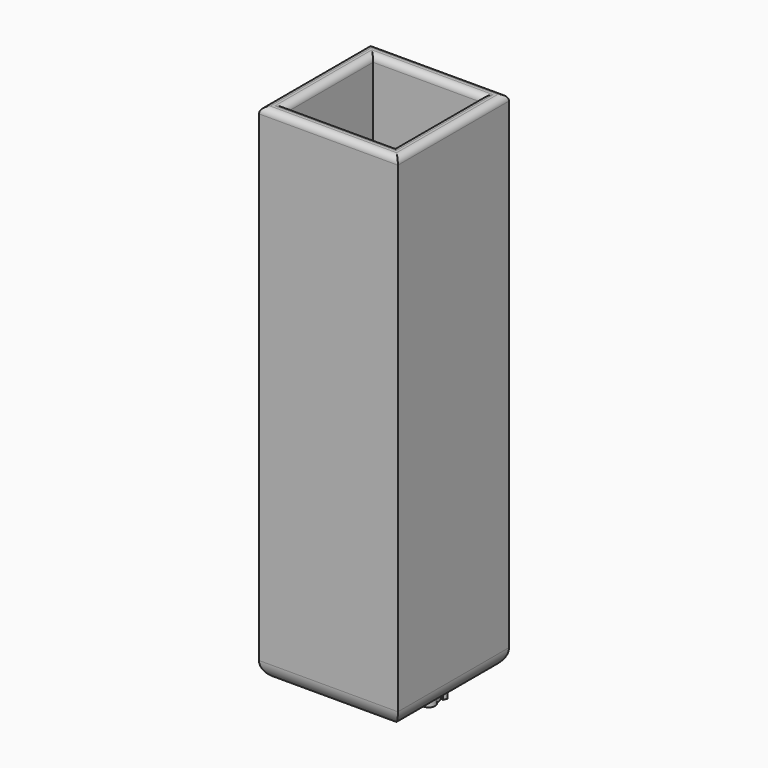
from build123d import *

# Parameters (mm, degrees)
F0_W         = 11
F0_H         = 11
F1_DEPTH     = 40
F2_W         = 8.6
F2_H         = 8.6
F3_DEPTH     = 25
F4_R         = 0.5
F5_R         = 1.4
F6_R         = 2
F7_TEXT_SIZE = 2.6055979644
F8_DEPTH     = 1


# Not quite as in the source:
# - Text() gives the source's letters only with a copy of the font that has no kerning and outlines rounded to 1/6400 em; it was checked with that copy


with BuildPart() as f1:
    # F0 (on Top) → F1 (new body)
    with BuildSketch(Plane.XY):
        Rectangle(F0_W, F0_H)
    extrude(amount=F1_DEPTH)

    # F2 (on face) → F3 (cut)
    with BuildSketch(Plane.XY.offset(40)):
        Rectangle(F2_W, F2_H)
    extrude(amount=-F3_DEPTH, mode=Mode.SUBTRACT)

    # F4
    f4_edges = [f1.edges().sort_by_distance(p)[0] for p in [
        (0, 5.5, 40),
        (5.5, 0, 40),
        (-5.5, 0, 40),
        (0, -5.5, 40),
        (0, -4.3, 40),
        (4.3, 0, 40),
        (0, 4.3, 40),
        (-4.3, 0, 40),
    ]]
    fillet(f4_edges, radius=F4_R)

    # F5
    f5_edges = [f1.edges().sort_by_distance(p)[0] for p in [
        (0, 5.5, 0),
        (-5.5, 0, 0),
        (0, -5.5, 0),
        (5.5, 0, 0),
    ]]
    fillet(f5_edges, radius=F5_R)

    # F6
    f6_edges = [f1.edges().sort_by_distance(p)[0] for p in [
        (0, -4.3, 15),
        (4.3, 0, 15),
        (0, 4.3, 15),
        (-4.3, 0, 15),
    ]]
    fillet(f6_edges, radius=F6_R)


with BuildPart() as f8:
    # F7 (on Top) → F8 (new body)
    with BuildSketch(Plane.XY):
        with Locations((-3.9, -0.3760305344)):
            Text('CiQUS', F7_TEXT_SIZE, font='Open Sans', font_style=FontStyle.BOLD, text_align=(TextAlign.LEFT, TextAlign.BOTTOM))
    extrude(amount=-F8_DEPTH)


with BuildPart() as f9_1:
    # F9: instance of F8
    add(f8.part.mirror(Plane.YZ))


solid = Compound([f1.part, f8.part, f9_1.part])
